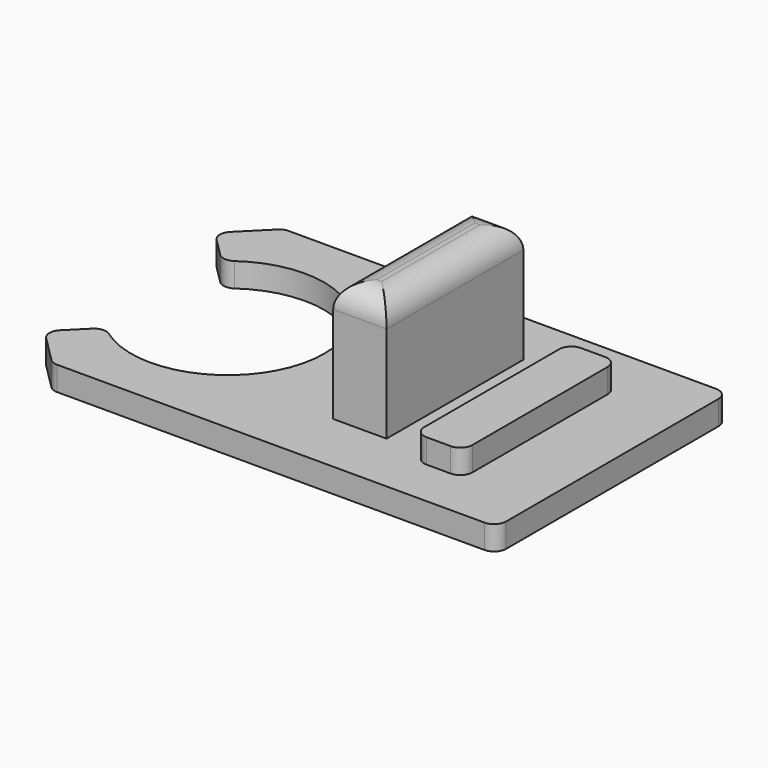
from build123d import *

# Parameters (mm, degrees)
F1_DEPTH = 1
F2_W     = 2
F2_H     = 8
F3_DEPTH = 1
F4_R     = 0.5
F5_W     = 2.2095986642
F5_H     = 7.0855088998
F6_DEPTH = 5
F7_R     = 1


with BuildPart() as f1:
    # F0 (on Top) → F1 (new body)
    with BuildSketch(Plane.XY):
        with BuildLine():
            ThreePointArc((-2.6457513111, 3), (4, 0), (-2.6457513111, -3))
            Line((-2.6457513111, -3), (-4.0599648734, -4.4142135624))
            Line((-4.0599648734, -4.4142135624), (-2.4741784358, -6))
            Line((-2.4741784358, -6), (15.9400351266, -6))
            Line((15.9400351266, -6), (15.9400351266, 6))
            Line((15.9400351266, 6), (-2.4741784358, 6))
            Line((-2.4741784358, 6), (-4.0599648734, 4.4142135624))
            Line((-4.0599648734, 4.4142135624), (-2.6457513111, 3))
        make_face()
    extrude(amount=F1_DEPTH)

    # F2 (on face) → F3 (join)
    with BuildSketch(Plane.XY.offset(1)):
        with Locations((11.9400351266, 0)):
            Rectangle(F2_W, F2_H)
    extrude(amount=F3_DEPTH)

    # F4
    f4_edges = [f1.edges().sort_by_distance(p)[0] for p in [
        (-2.645751, -3, 0.5),
        (-2.645751, 3, 0.5),
        (-4.059965, -4.414214, 0.5),
        (-2.474178, -6, 0.5),
        (-4.059965, 4.414214, 0.5),
        (-2.474178, 6, 0.5),
        (10.940035, -4, 1.5),
        (12.940035, -4, 1.5),
        (10.940035, 4, 1.5),
        (12.940035, 4, 1.5),
        (15.940035, 6, 0.5),
        (15.940035, -6, 0.5),
    ]]
    fillet(f4_edges, radius=F4_R)

    # F5 (on face) → F6 (join)
    with BuildSketch(Plane.XY.offset(1)):
        with Locations((8.1892169546, 0.1541808015)):
            Rectangle(F5_W, F5_H)
    extrude(amount=F6_DEPTH)

    # F7
    f7_edges = [f1.edges().sort_by_distance(p)[0] for p in [
        (8.189217, 3.696935, 6),
        (7.084418, 0.154181, 6),
        (8.189217, -3.388574, 6),
        (9.294016, 0.154181, 6),
    ]]
    fillet(f7_edges, radius=F7_R)


solid = f1.part
